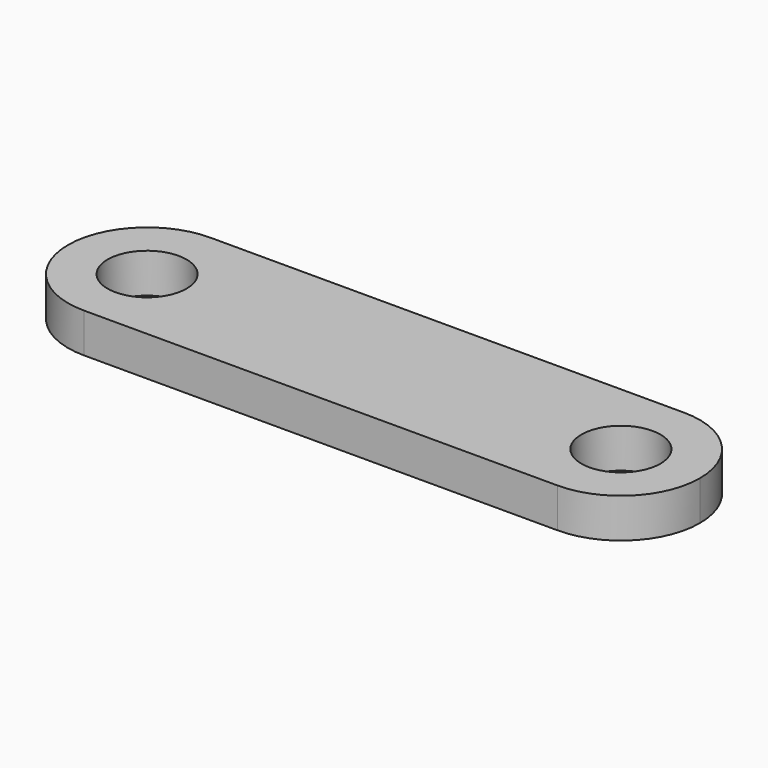
from build123d import *

# Parameters (mm, degrees)
F0_W          = 101.6
F0_H          = 25.4
F1_DEPTH      = 3.175
F1_DEPTH_BACK = 3.175
F2_R          = 6.35
F3_DEPTH      = 6.351
F4_DEPTH      = 6.351
F5_R          = 12.69999


# Not quite as in the source:
# - a fillet or chamfer is up to 0.001 mm smaller than in the source, because OpenCascade refuses the exact size


with BuildPart() as f1:
    # F0 (on Top) → F1 (new body, two sides)
    with BuildSketch(Plane.XY) as f1_sk:
        Rectangle(F0_W, F0_H)
    extrude(amount=F1_DEPTH)
    extrude(f1_sk.sketch, amount=-F1_DEPTH_BACK)

    # F2 (on face) → F3 (cut, through all)
    with BuildSketch(Plane.XY.offset(3.175)):
        with Locations((38.1, 0)):
            Circle(F2_R)
        with Locations((-38.1, 0)):
            Circle(F2_R)
    extrude(amount=-F3_DEPTH, mode=Mode.SUBTRACT)

    # F2 (on face) → F4 (cut, through all)
    with BuildSketch(Plane.XY.offset(3.175)):
        with Locations((38.1, 0)):
            Circle(F2_R)
        with Locations((-38.1, 0)):
            Circle(F2_R)
    extrude(amount=-F4_DEPTH, mode=Mode.SUBTRACT)

    # F5 (radius 12.7 in the source; OpenCascade refuses exactly that, so slightly less here)
    f5_edges = [f1.edges().sort_by_distance(p)[0] for p in [
        (50.8, -12.7, 0),
        (-50.8, -12.7, 0),
        (50.8, 12.7, 0),
        (-50.8, 12.7, 0),
    ]]
    fillet(f5_edges, radius=F5_R)


solid = f1.part
